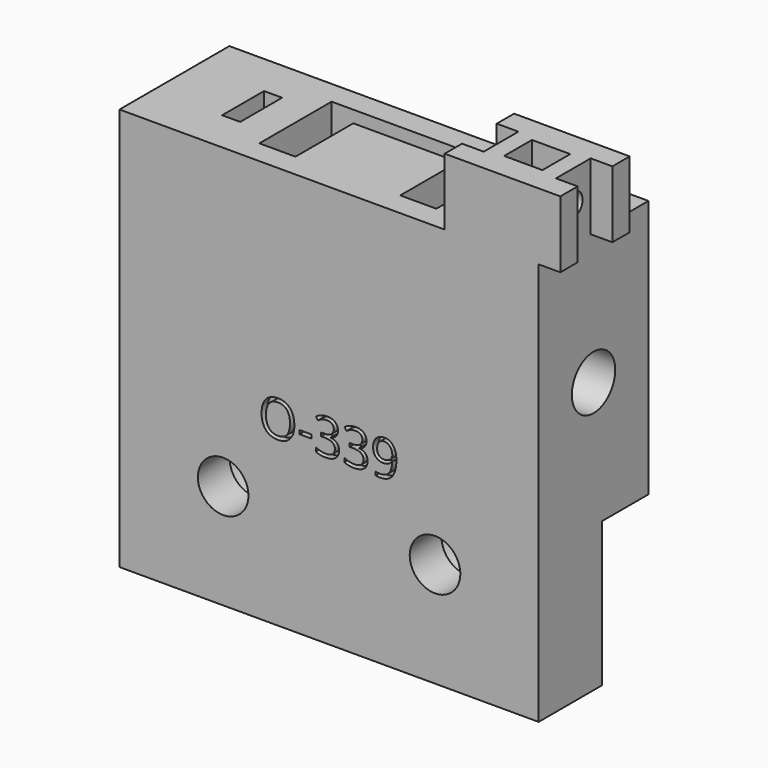
from build123d import *

# Parameters (mm, degrees)
F0_W          = 58
F0_H          = 19
F1_DEPTH      = 11
F2_W          = 58
F2_H          = 19
F3_DEPTH      = 24.75
F4_W          = 5
F4_H          = 12.5
F5_DEPTH      = 24.75
F6_R          = 2.25
F7_DEPTH      = 58.001
F8_W          = 14.5
F8_H          = 2.5
F9_DEPTH      = 24.75
F10_R         = 3.75
F11_DEPTH     = 10.75
F12_W         = 2.5
F12_H         = 7.25
F13_DEPTH     = 22
F14_TEXT_SIZE = 6.9078950522
F15_DEPTH     = 1
F17_DEPTH     = 9.25
F18_R         = 1.6
F19_DEPTH     = 13.0010001
F20_W         = 5.3
F20_H         = 4.8
F21_DEPTH     = 7
F22_W         = 58
F22_H         = 20
F23_DEPTH     = 11
F24_R         = 3.5
F25_DEPTH     = 11.0010001
F26_R         = 5.5
F27_DEPTH     = 5.5


# Not quite as in the source:
# - Text() gives the source's letters only with a copy of the font that has no kerning and outlines rounded to 1/6400 em; it was checked with that copy


with BuildPart() as f1:
    # F0 (on Top) → F1 (new body)
    with BuildSketch(Plane.XY):
        Rectangle(F0_W, F0_H)
    extrude(amount=F1_DEPTH)

    # F2 (on face) → F3 (join)
    with BuildSketch(Plane.XY.offset(11)):
        Rectangle(F2_W, F2_H)
    extrude(amount=F3_DEPTH)

    # F4 (on face) → F5 (cut)
    with BuildSketch(Plane.XY.offset(35.75)):
        with Locations((-9.75, 0)):
            Rectangle(F4_W, F4_H)
        with Locations((9.75, 0)):
            Rectangle(F4_W, F4_H)
    extrude(amount=-F5_DEPTH, mode=Mode.SUBTRACT)

    # F6 (on face) → F7 (cut, through all)
    with BuildSketch(Plane.YZ.offset(29)):
        with Locations((0, 17.5)):
            Circle(F6_R)
    extrude(amount=-F7_DEPTH, mode=Mode.SUBTRACT)

    # F8 (on face) → F9 (cut)
    with BuildSketch(Plane.XY.offset(35.75)):
        with Locations((0, 5)):
            Rectangle(F8_W, F8_H)
    extrude(amount=-F9_DEPTH, mode=Mode.SUBTRACT)

    # F10 (on face) → F11 (cut)
    with BuildSketch(Plane.YZ.offset(29)):
        with Locations((0, 17.5)):
            Circle(F10_R)
    extrude(amount=-F11_DEPTH, mode=Mode.SUBTRACT)

    # F12 (on face) → F13 (cut)
    with BuildSketch(Plane.XY.offset(35.75)):
        with Locations((-18.25, 0)):
            Rectangle(F12_W, F12_H)
    extrude(amount=-F13_DEPTH, mode=Mode.SUBTRACT)

    # F14 (on face) → F15 (cut)
    with BuildSketch(Plane.XZ.offset(9.5)):
        with Locations((-9.7638779128, 2.6940791868)):
            Text('O-339', F14_TEXT_SIZE, font='Open Sans', text_align=(TextAlign.LEFT, TextAlign.BOTTOM))
    extrude(amount=-F15_DEPTH, mode=Mode.SUBTRACT)

    # F16 (on face) → F17 (join)
    with BuildSketch(Plane.XY.offset(35.75)):
        Polygon((29, -6.5), (29, -0.5), (32, -0.5), (32, 2.5), (16, 2.5), (16, -0.5), (19, -0.5), (19, -6.5), (16, -6.5), (16, -9.5), (32, -9.5), (32, -6.5), align=None)
    extrude(amount=F17_DEPTH)

    # F18 (on face) → F19 (cut, through all)
    with BuildSketch(Plane(origin=(19, 0, 0), x_dir=(0, -1, 0), z_dir=(-1, 0, 0))):
        with Locations((3.5, 40.5616685748)):
            Circle(F18_R)
    extrude(amount=-F19_DEPTH, mode=Mode.SUBTRACT)

    # F20 (on face) → F21 (cut)
    with BuildSketch(Plane.XY.offset(45)):
        with Locations((24, -3.5)):
            Rectangle(F20_W, F20_H)
    extrude(amount=-F21_DEPTH, mode=Mode.SUBTRACT)

    # F22 (on face) → F23 (join)
    with BuildSketch(Plane.XZ.offset(9.5)):
        with Locations((0, -10)):
            Rectangle(F22_W, F22_H)
    extrude(amount=-F23_DEPTH)

    # F24 (on face) → F25 (cut, through all)
    with BuildSketch(Plane(origin=(0, 1.5, 0), x_dir=(-1, 0, 0), z_dir=(0, 1, 0))):
        with Locations((-14.6586513147, -5.5)):
            Circle(F24_R)
        with Locations((14.6586513147, -5.5)):
            Circle(F24_R)
    extrude(amount=-F25_DEPTH, mode=Mode.SUBTRACT)

    # F26 (on face) → F27 (cut)
    with BuildSketch(Plane(origin=(0, 1.5, 0), x_dir=(-1, 0, 0), z_dir=(0, 1, 0))):
        with Locations((-14.6586513147, -5.5)):
            Circle(F26_R)
        with Locations((14.6586513147, -5.5)):
            Circle(F26_R)
    extrude(amount=-F27_DEPTH, mode=Mode.SUBTRACT)


solid = f1.part
